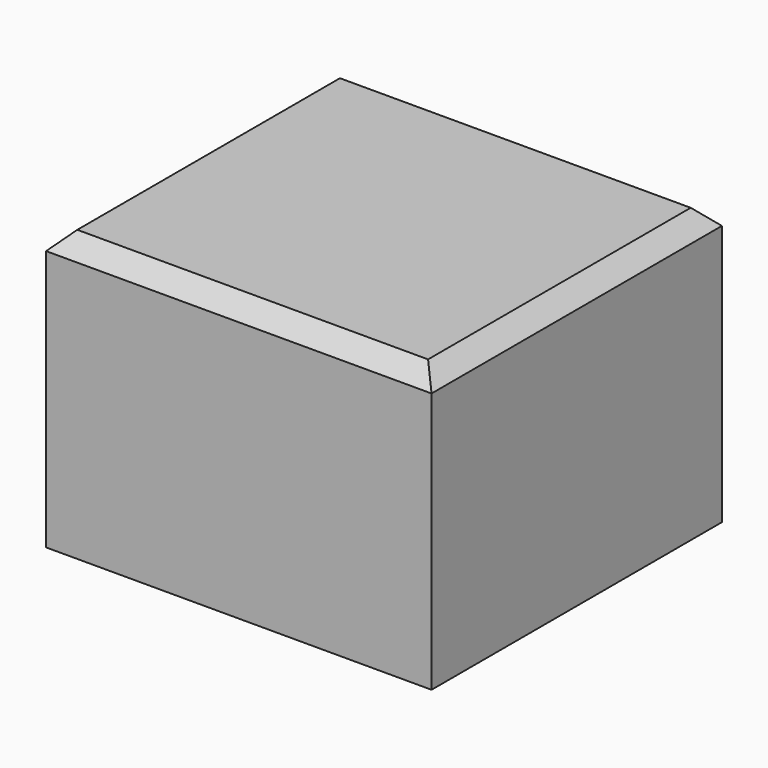
from build123d import *

# Parameters (mm, degrees)
F0_W     = 112.9649430513
F0_H     = 106.3782721758
F1_DEPTH = 81.534
F2_SIZE  = 5.08


# Not quite as in the source:
# - a feature of the source that left no trace in its solid (it failed there, or was rolled back) is left out


with BuildPart() as f1:
    # F0 (on Top) → F1 (new body)
    with BuildSketch(Plane.XY):
        with Locations((-18.7927857041, -9.1543830931)):
            Rectangle(F0_W, F0_H)
    extrude(amount=F1_DEPTH)

    # F2
    f2_edges = [f1.edges().sort_by_distance(p)[0] for p in [
        (-18.792786, 44.034753, 81.534),
        (-75.275257, -9.154383, 81.534),
        (-18.792786, -62.343519, 81.534),
        (37.689686, -9.154383, 81.534),
    ]]
    chamfer(f2_edges, length=F2_SIZE)


solid = f1.part
